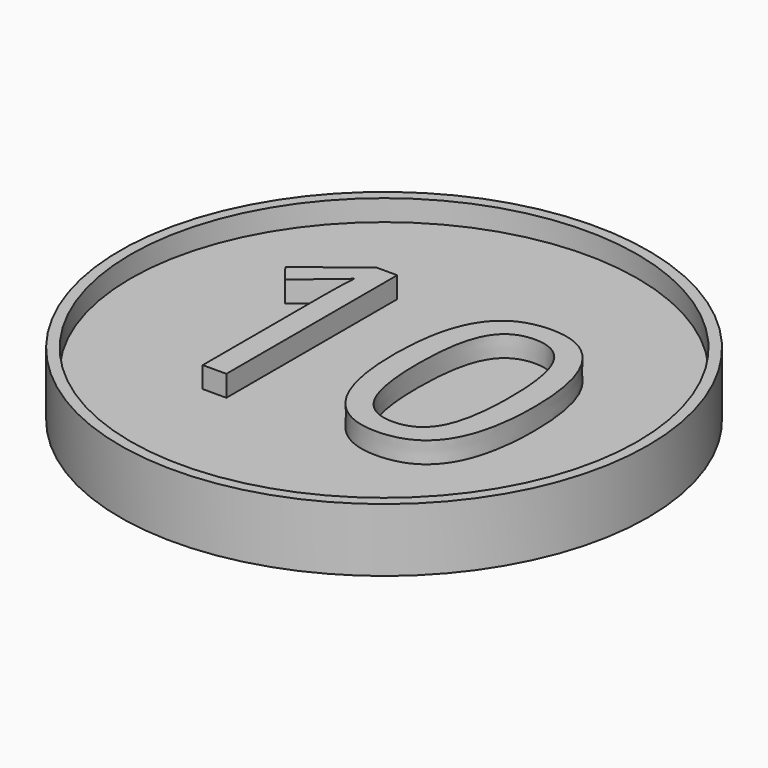
from build123d import *

# Parameters (mm, degrees)
F2_R         = 12.5
F3_DEPTH     = 3
F4_R         = 12
F5_DEPTH     = 1
F6_R         = 12
F7_DEPTH     = 1
F8_TEXT_SIZE = 14.1666666667
F9_DEPTH     = 1


# Not quite as in the source:
# - Text() gives the source's letters only with a copy of the font that has no kerning and outlines rounded to 1/6400 em; it was checked with that copy


with BuildPart() as f3:
    # F2 (on Top) → F3 (new body)
    with BuildSketch(Plane.XY):
        with Locations((0, 0.1589417938)):
            Circle(F2_R)
    extrude(amount=F3_DEPTH)

    # F4 (on face) → F5 (cut)
    with BuildSketch(Plane.XY.offset(3)):
        with Locations((0, 0.1589417938)):
            Circle(F4_R)
    extrude(amount=-F5_DEPTH, mode=Mode.SUBTRACT)

    # F6 (on face) → F7 (cut)
    with BuildSketch(Plane(origin=(0, 0, 0), x_dir=(1, 0, 0), z_dir=(0, 0, -1))):
        with Locations((0, -0.1589417938)):
            Circle(F6_R)
    extrude(amount=-F7_DEPTH, mode=Mode.SUBTRACT)

    # F8 (on face) → F9 (join)
    with BuildSketch(Plane.XY.offset(2)):
        with Locations((-8.2067057292, -5.1)):
            Text('10', F8_TEXT_SIZE, font='Open Sans', text_align=(TextAlign.LEFT, TextAlign.BOTTOM))
    extrude(amount=F9_DEPTH)


solid = f3.part
